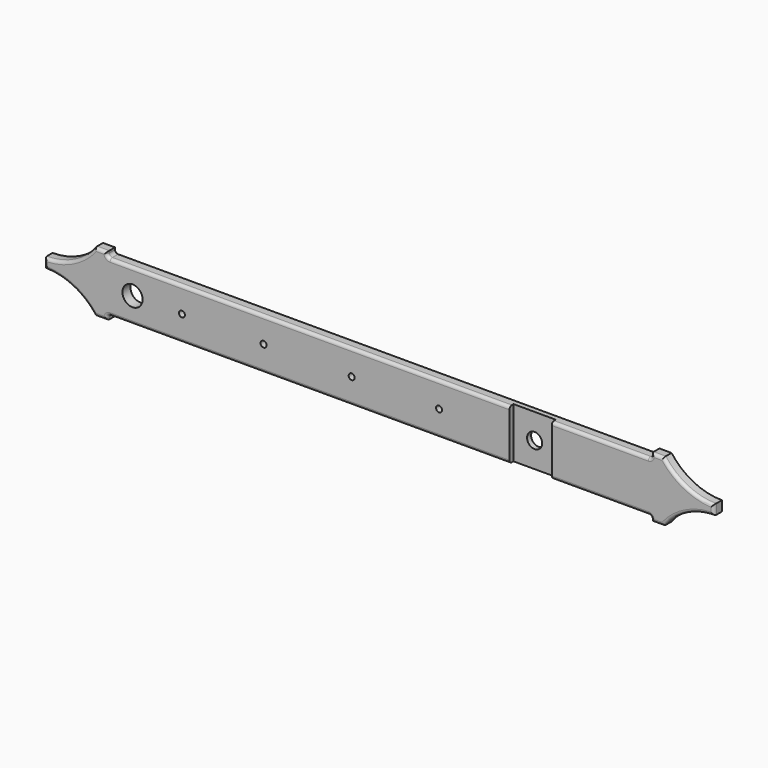
from build123d import *

# Parameters (mm, degrees)
F0_R         = 10
F0_R_2       = 3
F0_R_3       = 7.5
F1_DEPTH     = 10
F2_W         = 42
F2_H         = 50
F2_R         = 7.5
F3_DEPTH     = 5
F4_T1_DEPTH  = 403.7
F4_T3_DEPTH  = 103.3
F4_T5_DEPTH  = 27
F4_T7_DEPTH  = 25
F4_T9_DEPTH  = 27
F4_T11_DEPTH = 9.5
F4_T13_DEPTH = 9.5
F4_T16_ANGLE = 66.8830141294
F4_T18_ANGLE = 66.8830141294
F4_T20_ANGLE = 66.8830141294
F4_T22_ANGLE = 66.8830141294
F4_T24_ANGLE = 90
F4_T26_ANGLE = 90
F4_T28_ANGLE = 90
F4_T30_ANGLE = 90


# Not quite as in the source:
# - a fillet or chamfer that OpenCascade refuses, or shapes differently, is made with other operations: its cross-section is extruded or revolved along the edge and cut away or added


with BuildPart() as f1:
    # F0 (on Front) → F1 (new body)
    with BuildSketch(Plane.XZ):
        with BuildLine():
            Line((0, -5), (0, 0))
            Line((0, 0), (0, 5))
            ThreePointArc((0, 5), (-27.9508497187, 11.5983005625), (-50, 30))
            Line((-50, 30), (-62, 30))
            Line((-62, 30), (-62, 28))
            ThreePointArc((-62, 28), (-62.8786796564, 25.8786796564), (-65, 25))
            Line((-65, 25), (-332, 25))
            Line((-332, 25), (-599, 25))
            ThreePointArc((-599, 25), (-601.1213203436, 25.8786796564), (-602, 28))
            Line((-602, 28), (-602, 30))
            Line((-602, 30), (-614, 30))
            ThreePointArc((-614, 30), (-636.0491502813, 11.5983005625), (-664, 5))
            Line((-664, 5), (-664, 0))
            Line((-664, 0), (-664, -5))
            ThreePointArc((-664, -5), (-636.0491502813, -11.5983005625), (-614, -30))
            Line((-614, -30), (-602, -30))
            Line((-602, -30), (-602, -28))
            ThreePointArc((-602, -28), (-601.1213203436, -25.8786796564), (-599, -25))
            Line((-599, -25), (-332, -25))
            Line((-332, -25), (-65, -25))
            ThreePointArc((-65, -25), (-62.8786796564, -25.8786796564), (-62, -28))
            Line((-62, -28), (-62, -30))
            Line((-62, -30), (-50, -30))
            ThreePointArc((-50, -30), (-27.9508497187, -11.5983005625), (0, -5))
        make_face()
        with Locations((-576.7, 0)):
            Circle(F0_R, mode=Mode.SUBTRACT)
        with Locations((-527.7, 0)):
            Circle(F0_R_2, mode=Mode.SUBTRACT)
        with Locations((-446.7, 0)):
            Circle(F0_R_2, mode=Mode.SUBTRACT)
        with Locations((-359.3, 0)):
            Circle(F0_R_2, mode=Mode.SUBTRACT)
        with Locations((-272.6, 0)):
            Circle(F0_R_2, mode=Mode.SUBTRACT)
        with Locations((-181.8, 0)):
            Circle(F0_R_3, mode=Mode.SUBTRACT)
    extrude(amount=F1_DEPTH)

    # F2 (on face) → F3 (cut)
    with BuildSketch(Plane.XZ.offset(10)):
        with Locations((-181.8, 0)):
            Rectangle(F2_W, F2_H)
        with Locations((-181.8, 0)):
            Circle(F2_R, mode=Mode.SUBTRACT)
    extrude(amount=-F3_DEPTH, mode=Mode.SUBTRACT)

    # F4: fillet of radius 3 on 18 edges, made by hand

    # F4_s2 → F4_t1 (cut)
    with BuildSketch(Plane.YZ.offset(-599)):
        with BuildLine():
            ThreePointArc((-10, 22), (-9.1213203436, 24.1213203436), (-7, 25))
            Line((-7, 25), (-10, 25))
            Line((-10, 25), (-10, 22))
        make_face()
        with BuildLine():
            ThreePointArc((-7, -25), (-9.1213203436, -24.1213203436), (-10, -22))
            Line((-10, -22), (-10, -25))
            Line((-10, -25), (-7, -25))
        make_face()
    extrude(amount=F4_T1_DEPTH, mode=Mode.SUBTRACT)

    # F4_s4 → F4_t3 (cut)
    with BuildSketch(Plane.YZ.offset(-168.3)):
        with BuildLine():
            ThreePointArc((-7, -25), (-9.1213203436, -24.1213203436), (-10, -22))
            Line((-10, -22), (-10, -25))
            Line((-10, -25), (-7, -25))
        make_face()
        with BuildLine():
            ThreePointArc((-10, 22), (-9.1213203436, 24.1213203436), (-7, 25))
            Line((-7, 25), (-10, 25))
            Line((-10, 25), (-10, 22))
        make_face()
    extrude(amount=F4_T3_DEPTH, mode=Mode.SUBTRACT)

    # F4_s6 → F4_t5 (cut)
    with BuildSketch(Plane.YZ.offset(-69.5)):
        with BuildLine():
            ThreePointArc((-10, -27), (-9.1213203436, -29.1213203436), (-7, -30))
            Line((-7, -30), (-10, -30))
            Line((-10, -30), (-10, -27))
        make_face()
        with BuildLine():
            ThreePointArc((-10, 27), (-9.1213203436, 29.1213203436), (-7, 30))
            Line((-7, 30), (-10, 30))
            Line((-10, 30), (-10, 27))
        make_face()
    extrude(amount=F4_T5_DEPTH, mode=Mode.SUBTRACT)

    # F4_s8 → F4_t7 (cut)
    with BuildSketch(Plane.XY.offset(-12.5)):
        with BuildLine():
            ThreePointArc((-3, -10), (-0.8786796564, -9.1213203436), (0, -7))
            Line((0, -7), (0, -10))
            Line((0, -10), (-3, -10))
        make_face()
        with BuildLine():
            ThreePointArc((-661, -10), (-663.1213203436, -9.1213203436), (-664, -7))
            Line((-664, -7), (-664, -10))
            Line((-664, -10), (-661, -10))
        make_face()
    extrude(amount=F4_T7_DEPTH, mode=Mode.SUBTRACT)

    # F4_s10 → F4_t9 (cut)
    with BuildSketch(Plane.YZ.offset(-621.5)):
        with BuildLine():
            ThreePointArc((-10, -27), (-9.1213203436, -29.1213203436), (-7, -30))
            Line((-7, -30), (-10, -30))
            Line((-10, -30), (-10, -27))
        make_face()
        with BuildLine():
            ThreePointArc((-10, 27), (-9.1213203436, 29.1213203436), (-7, 30))
            Line((-7, 30), (-10, 30))
            Line((-10, 30), (-10, 27))
        make_face()
    extrude(amount=F4_T9_DEPTH, mode=Mode.SUBTRACT)

    # F4_s12 → F4_t11 (cut)
    with BuildSketch(Plane.XY.offset(28)):
        with BuildLine():
            ThreePointArc((-605, -10), (-602.8786796564, -9.1213203436), (-602, -7))
            Line((-602, -7), (-602, -10))
            Line((-602, -10), (-605, -10))
        make_face()
        with BuildLine():
            ThreePointArc((-59, -10), (-61.1213203436, -9.1213203436), (-62, -7))
            Line((-62, -7), (-62, -10))
            Line((-62, -10), (-59, -10))
        make_face()
    extrude(amount=F4_T11_DEPTH, mode=Mode.SUBTRACT)

    # F4_s14 → F4_t13 (cut)
    with BuildSketch(Plane.XY.offset(-37.5)):
        with BuildLine():
            ThreePointArc((-605, -10), (-602.8786796564, -9.1213203436), (-602, -7))
            Line((-602, -7), (-602, -10))
            Line((-602, -10), (-605, -10))
        make_face()
        with BuildLine():
            ThreePointArc((-59, -10), (-61.1213203436, -9.1213203436), (-62, -7))
            Line((-62, -7), (-62, -10))
            Line((-62, -10), (-59, -10))
        make_face()
    extrude(amount=F4_T13_DEPTH, mode=Mode.SUBTRACT)

    # F4_s15 → F4_t16 (revolve, cut)
    with BuildSketch(Plane(origin=(-29.2244934886, 0, -50.6316906835), x_dir=(0, 1, 0), z_dir=(-0.4999008689, 0, -0.8660826296))):
        with BuildLine():
            ThreePointArc((-10, -31.7566913469), (-9.1213203436, -29.6353710033), (-7, -28.7566913469))
            Line((-7, -28.7566913469), (-10, -28.7566913469))
            Line((-10, -28.7566913469), (-10, -31.7566913469))
        make_face()
    revolve(axis=Axis((0, -10, -67.5), (0, 1, 0)), revolution_arc=F4_T16_ANGLE, mode=Mode.SUBTRACT)

    # F4_s17 → F4_t18 (revolve, cut)
    with BuildSketch(Plane(origin=(8.0235648794, 0, 0.9676128596), x_dir=(0, 1, 0), z_dir=(0.992806625, 0, 0.1197288826))):
        with BuildLine():
            ThreePointArc((-10, 1.5144471885), (-9.1213203436, 3.6357675321), (-7, 4.5144471885))
            Line((-7, 4.5144471885), (-10, 4.5144471885))
            Line((-10, 4.5144471885), (-10, 1.5144471885))
        make_face()
    revolve(axis=Axis((0, -10, 67.5), (0, 1, 0)), revolution_arc=F4_T18_ANGLE, mode=Mode.SUBTRACT)

    # F4_s19 → F4_t20 (revolve, cut)
    with BuildSketch(Plane(origin=(-662.5051213425, 0, -79.8957177472), x_dir=(0, 1, 0), z_dir=(-0.992806625, 0, -0.1197288826))):
        with BuildLine():
            ThreePointArc((-10, -77.9855308525), (-9.1213203436, -75.864210509), (-7, -74.9855308525))
            Line((-7, -74.9855308525), (-10, -74.9855308525))
            Line((-10, -74.9855308525), (-10, -77.9855308525))
        make_face()
    revolve(axis=Axis((-664, -10, -67.5), (0, 1, 0)), revolution_arc=F4_T20_ANGLE, mode=Mode.SUBTRACT)

    # F4_s21 → F4_t22 (revolve, cut)
    with BuildSketch(Plane(origin=(-136.7096900096, 0, -236.8507341524), x_dir=(0, 1, 0), z_dir=(0.4999008689, 0, 0.8660826296))):
        with BuildLine():
            ThreePointArc((-10, 543.3221746856), (-9.1213203436, 545.4434950292), (-7, 546.3221746856))
            Line((-7, 546.3221746856), (-10, 546.3221746856))
            Line((-10, 546.3221746856), (-10, 543.3221746856))
        make_face()
    revolve(axis=Axis((-664, -10, 67.5), (0, 1, 0)), revolution_arc=F4_T22_ANGLE, mode=Mode.SUBTRACT)

    # F4_s23 → F4_t24 (revolve, cut)
    with BuildSketch(Plane.YZ.offset(-65)):
        with BuildLine():
            ThreePointArc((-7, -25), (-9.1213203436, -24.1213203436), (-10, -22))
            Line((-10, -22), (-10, -25))
            Line((-10, -25), (-7, -25))
        make_face()
    revolve(axis=Axis((-65, -10, -28), (0, 1, 0)), revolution_arc=F4_T24_ANGLE, mode=Mode.SUBTRACT)

    # F4_s25 → F4_t26 (revolve, cut)
    with BuildSketch(Plane.XY.offset(28)):
        with BuildLine():
            ThreePointArc((-59, -10), (-61.1213203436, -9.1213203436), (-62, -7))
            Line((-62, -7), (-62, -10))
            Line((-62, -10), (-59, -10))
        make_face()
    revolve(axis=Axis((-65, -10, 28), (0, 1, 0)), revolution_arc=F4_T26_ANGLE, mode=Mode.SUBTRACT)

    # F4_s27 → F4_t28 (revolve, cut)
    with BuildSketch(Plane.XY.offset(-28)):
        with BuildLine():
            ThreePointArc((-605, -10), (-602.8786796564, -9.1213203436), (-602, -7))
            Line((-602, -7), (-602, -10))
            Line((-602, -10), (-605, -10))
        make_face()
    revolve(axis=Axis((-599, -10, -28), (0, 1, 0)), revolution_arc=F4_T28_ANGLE, mode=Mode.SUBTRACT)

    # F4_s29 → F4_t30 (revolve, cut)
    with BuildSketch(Plane.YZ.offset(-599)):
        with BuildLine():
            ThreePointArc((-10, 22), (-9.1213203436, 24.1213203436), (-7, 25))
            Line((-7, 25), (-10, 25))
            Line((-10, 25), (-10, 22))
        make_face()
    revolve(axis=Axis((-599, -10, 28), (0, 1, 0)), revolution_arc=F4_T30_ANGLE, mode=Mode.SUBTRACT)


solid = f1.part
